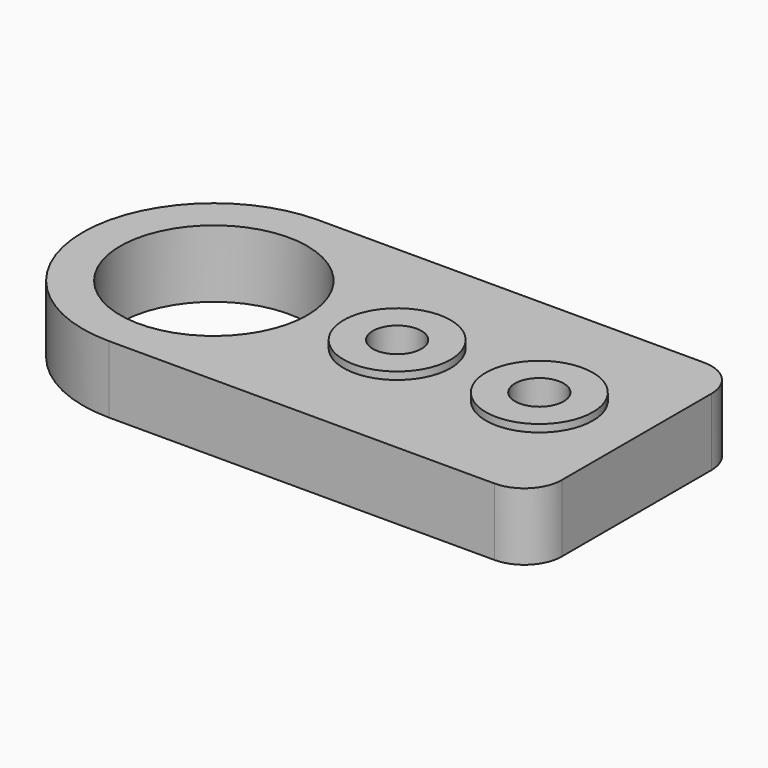
from build123d import *

# Parameters (mm, degrees)
F0_R         = 12.5
F1_DEPTH     = 9
F2_R         = 7.15
F2_R_2       = 3.25
F3_DEPTH     = 1
F4_DEPTH     = 8
F5_TEXT_SIZE = 5.5555555556
F6_DEPTH     = 1


# Not quite as in the source:
# - Text() gives the source's letters only with a copy of the font that has no kerning and outlines rounded to 1/6400 em; it was checked with that copy


with BuildPart() as f1:
    # F0 (on Top) → F1 (new body)
    with BuildSketch(Plane.XY):
        with BuildLine():
            ThreePointArc((0, 17.5), (5.1256313292, 5.1256313292), (17.5, 0))
            Line((17.5, 0), (69, 0))
            ThreePointArc((69, 0), (72.5355339059, 1.4644660941), (74, 5))
            Line((74, 5), (74, 30))
            ThreePointArc((74, 30), (72.5355339059, 33.5355339059), (69, 35))
            Line((69, 35), (17.5, 35))
            ThreePointArc((17.5, 35), (5.1256313292, 29.8743686708), (0, 17.5))
        make_face()
        with Locations((17.5, 17.5)):
            Circle(F0_R, mode=Mode.SUBTRACT)
    extrude(amount=F1_DEPTH)

    # F2 (on face) → F3 (join)
    with BuildSketch(Plane.XY.offset(9)):
        with Locations((42, 17.5)):
            Circle(F2_R)
        with Locations((42, 17.5)):
            Circle(F2_R_2, mode=Mode.SUBTRACT)
        with Locations((61, 17.5)):
            Circle(F2_R)
        with Locations((61, 17.5)):
            Circle(F2_R_2, mode=Mode.SUBTRACT)
    extrude(amount=F3_DEPTH)

    # F4 (cut): faces of the model
    f4_faces = [f1.faces().sort_by_distance(p)[0] for p in [
        (42, 17.5, 9),
        (61, 17.5, 9),
    ]]
    extrude(f4_faces, amount=-F4_DEPTH, mode=Mode.SUBTRACT)

    # F5 (on face) → F6 (cut)
    with BuildSketch(Plane(origin=(0, 0, 0), x_dir=(1, 0, 0), z_dir=(0, 0, -1))):
        with Locations((30, -9)):
            Text('964', F5_TEXT_SIZE, font='Open Sans', text_align=(TextAlign.LEFT, TextAlign.BOTTOM))
    extrude(amount=-F6_DEPTH, mode=Mode.SUBTRACT)


solid = f1.part
